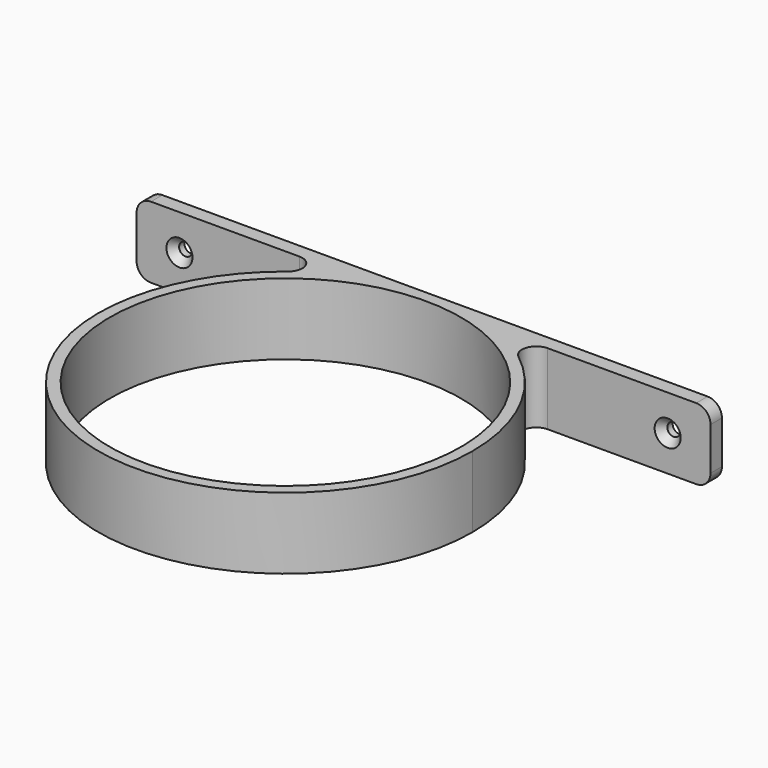
from build123d import *

# Parameters (mm, degrees)
F1_DEPTH       = 25
F2_R           = 5
F3_R           = 5
F5_D           = 4.4958
F5_DEPTH       = 5
F5_CSINK_D     = 9.1186
F5_CSINK_ANGLE = 82
F5_TIP         = 1.3506745855


with BuildPart() as f1:
    # F0 (on Top) → F1 (new body)
    with BuildSketch(Plane.XY):
        with BuildLine():
            ThreePointArc((65.5, -63), (54.4714923246, -26.6254687462), (25.099800796, -2.5))
            Line((25.099800796, -2.5), (11.0453610172, -2.5))
            ThreePointArc((11.0453610172, -2.5), (47.2310263627, -23.6111672079), (61.5, -63))
            ThreePointArc((61.5, -63), (-39.3888327921, -110.2310263627), (-11.0453610172, -2.5))
            Line((-11.0453610172, -2.5), (-25.099800796, -2.5))
            ThreePointArc((-25.099800796, -2.5), (-36.3745312538, -117.4714923246), (65.5, -63))
        make_face()
        with BuildLine():
            Line((0, 2.5), (-100.5, 2.5))
            Line((-100.5, 2.5), (-100.5, -2.5))
            Line((-100.5, -2.5), (-25.099800796, -2.5))
            ThreePointArc((-25.099800796, -2.5), (-12.7964838921, 1.2378393161), (0, 2.5))
        make_face()
        with BuildLine():
            ThreePointArc((25.099800796, -2.5), (12.7964838921, 1.2378393161), (0, 2.5))
            ThreePointArc((0, 2.5), (-12.7964838921, 1.2378393161), (-25.099800796, -2.5))
            Line((-25.099800796, -2.5), (-11.0453610172, -2.5))
            ThreePointArc((-11.0453610172, -2.5), (0, -1.5), (11.0453610172, -2.5))
            Line((11.0453610172, -2.5), (25.099800796, -2.5))
        make_face()
        with BuildLine():
            Line((100.5, 2.5), (0, 2.5))
            ThreePointArc((0, 2.5), (12.7964838921, 1.2378393161), (25.099800796, -2.5))
            Line((25.099800796, -2.5), (100.5, -2.5))
            Line((100.5, -2.5), (100.5, 2.5))
        make_face()
    extrude(amount=F1_DEPTH)

    # F2
    f2_edges = [f1.edges().sort_by_distance(p)[0] for p in [
        (-25.099801, -2.5, 12.5),
        (25.099801, -2.5, 12.5),
    ]]
    fillet(f2_edges, radius=F2_R)

    # F3
    f3_edges = [f1.edges().sort_by_distance(p)[0] for p in [
        (-100.5, 0, 25),
        (-100.5, 0, 0),
        (100.5, 0, 25),
        (100.5, 0, 0),
    ]]
    fillet(f3_edges, radius=F3_R)

    # F5
    with Locations(Plane.XZ.offset(2.5)):
        with Locations((-85.5, 12.5), (85.5, 12.5)):
            CounterSinkHole(F5_D / 2, F5_CSINK_D / 2, depth=F5_DEPTH, counter_sink_angle=F5_CSINK_ANGLE)
            with Locations((0, 0, -(F5_DEPTH + F5_TIP / 2))):  # 118° drill point
                Cone(0, F5_D / 2, F5_TIP, mode=Mode.SUBTRACT)


solid = f1.part
